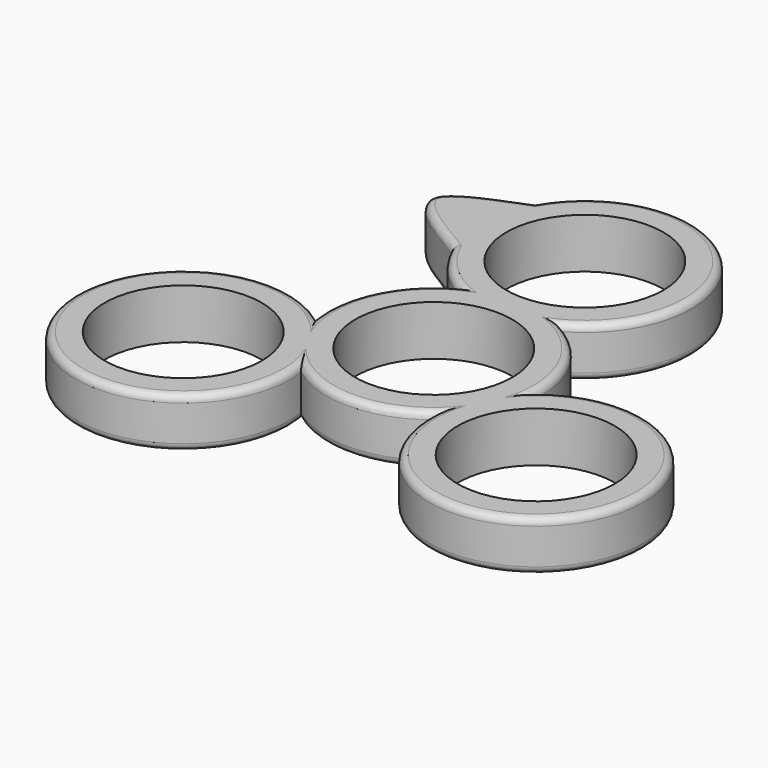
from build123d import *

# Parameters (mm, degrees)
F0_R     = 10.9855
F1_DEPTH = 7
F2_R     = 1
F4_R     = 1


# Not quite as in the source:
# - a feature of the source that left no trace in its solid (it failed there, or was rolled back) is left out


with BuildPart() as f1:
    # F0 (on Top) → F1 (new body)
    with BuildSketch(Plane.XY):
        with BuildLine():
            ThreePointArc((14.943845615, -1.1232427324), (13.1360253385, 7.2128381589), (7.0724560016, 13.2121369243))
            ThreePointArc((7.0724560016, 13.2121369243), (10.7716659316, 36.8430745981), (-12.9693349279, 33.9327056108))
            add(Edge.make_bspline(
                [(-12.9693349279, 33.9327056108), (-17.7567542547, 32.0721261538), (-27.5247485867, 28.3576089898), (-18.2844256096, 22.9473210363), (-13.6402039043, 20.2174201006)],
                knots=[0, 0, 0, 0, 0.4944320875, 1, 1, 1, 1], degree=3))
            ThreePointArc((-13.6402039043, 20.2174201006), (-10.9326148834, 16.1744871283), (-7.0724560016, 13.2121369243))
            ThreePointArc((-7.0724560016, 13.2121369243), (-13.3501998033, 6.808256841), (-14.8473809618, -2.0335866286))
            ThreePointArc((-14.8473809618, -2.0335866286), (-36.7528541273, -21.6235041555), (-8.9891687685, -11.9906230385))
            ThreePointArc((-8.9891687685, -11.9906230385), (0.3483794335, -14.9819500657), (9.5367940602, -11.5598336949))
            ThreePointArc((9.5367940602, -11.5598336949), (37.7868802207, -19.5768532256), (14.943845615, -1.1232427324))
        make_face()
        with Locations((-23.8365497302, -14.0242096671)):
            Circle(F0_R, mode=Mode.SUBTRACT)
        Circle(F0_R, mode=Mode.SUBTRACT)
        with Locations((24.4806396752, -12.6830764273)):
            Circle(F0_R, mode=Mode.SUBTRACT)
        with Locations((0, 26.4242738485)):
            Circle(F0_R, mode=Mode.SUBTRACT)
    extrude(amount=F1_DEPTH)

    # F2
    f2_edges = [f1.edges().sort_by_distance(p)[0] for p in [
        (10.771666, 36.843075, 7),
        (-22.76964, 27.719776, 7),
        (-10.932615, 16.174487, 7),
        (-13.3502, 6.808257, 7),
        (-36.752854, -21.623504, 7),
        (0.348379, -14.98195, 7),
        (37.78688, -19.576853, 7),
        (13.136025, 7.212838, 7),
    ]]
    fillet(f2_edges, radius=F2_R)

    # F4
    f4_edges = [f1.edges().sort_by_distance(p)[0] for p in [
        (37.78688, -19.576853, 0),
        (0.348379, -14.98195, 0),
        (-36.752854, -21.623504, 0),
        (-13.3502, 6.808257, 0),
        (-10.932615, 16.174487, 0),
        (13.136025, 7.212838, 0),
        (10.771666, 36.843075, 0),
        (-22.773556, 27.908211, 0),
    ]]
    fillet(f4_edges, radius=F4_R)


solid = f1.part
